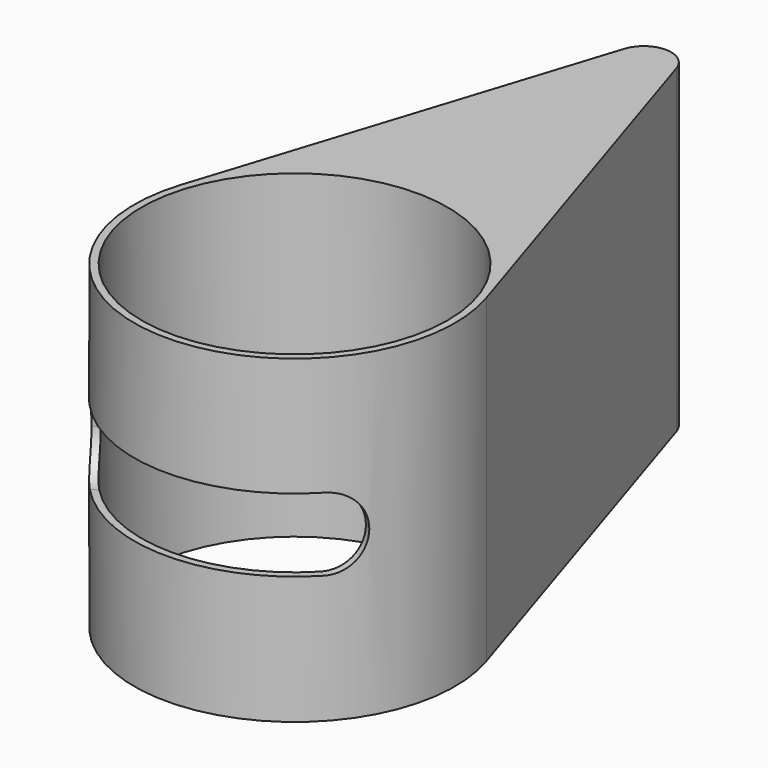
from build123d import *

# Parameters (mm, degrees)
F0_R          = 16.75
F1_DEPTH      = 17
F1_DEPTH_BACK = 18
F3_DEPTH      = 4
F3_DEPTH_BACK = 4
F4_R          = 3.99999


# Not quite as in the source:
# - a fillet or chamfer is up to 0.001 mm smaller than in the source, because OpenCascade refuses the exact size
# - a feature of the source that left no trace in its solid (it failed there, or was rolled back) is left out


with BuildPart() as f1:
    # F0 (on Top) → F1 (new body, two sides)
    with BuildSketch(Plane.XY) as f1_sk:
        with BuildLine():
            Line((-2.8573335724, 48.6641361257), (-16.7154013983, 5.3476963351))
            ThreePointArc((-16.7154013983, 5.3476963351), (0, -17.55), (16.7154013983, 5.3476963351))
            Line((16.7154013983, 5.3476963351), (2.8573335724, 48.6641361257))
            ThreePointArc((2.8573335724, 48.6641361257), (0, 50.75), (-2.8573335724, 48.6641361257))
        make_face()
        Circle(F0_R, mode=Mode.SUBTRACT)
    extrude(amount=F1_DEPTH)
    extrude(f1_sk.sketch, amount=-F1_DEPTH_BACK)

    # F2 (on Top) → F3 (cut, two sides)
    with BuildSketch(Plane.XY) as f3_sk:
        with BuildLine():
            Line((15.1987458364, -8.775), (0, 0))
            Line((0, 0), (-15.1987458364, -8.775))
            ThreePointArc((-15.1987458364, -8.775), (0, -17.55), (15.1987458364, -8.775))
        make_face()
    extrude(amount=F3_DEPTH, mode=Mode.SUBTRACT)
    extrude(f3_sk.sketch, amount=-F3_DEPTH_BACK, mode=Mode.SUBTRACT)

    # F4 (radius 4 in the source; OpenCascade refuses exactly that, so slightly less here)
    f4_edges = [f1.edges().sort_by_distance(p)[0] for p in [
        (-14.852336, -8.575, 4),
        (-14.852336, -8.575, -4),
        (14.852336, -8.575, -4),
        (14.852336, -8.575, 4),
    ]]
    fillet(f4_edges, radius=F4_R)


solid = f1.part
